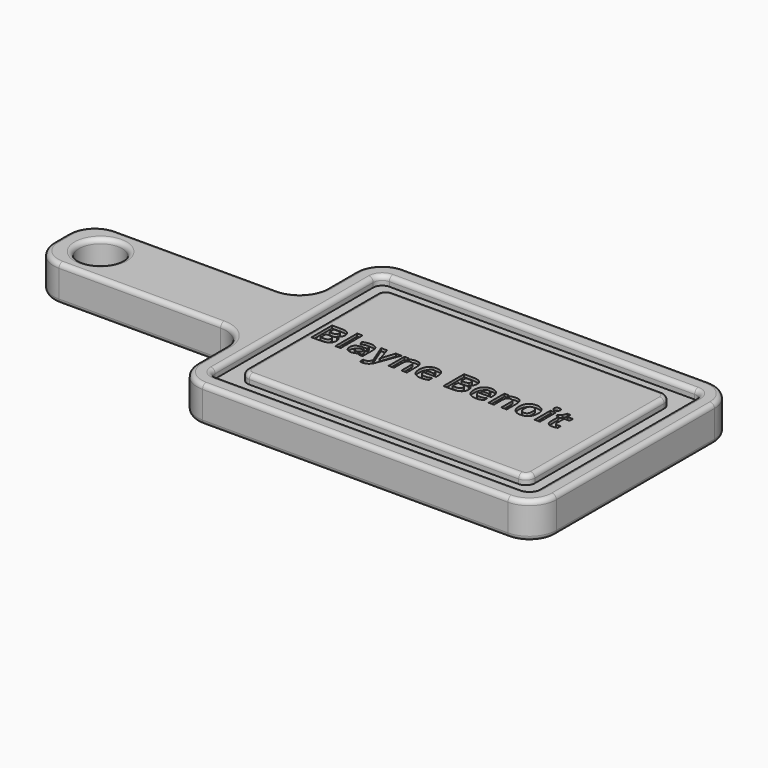
from build123d import *

# Parameters (mm, degrees)
F0_W         = 152.4
F0_H         = 50.8
F1_DEPTH     = 25.4
F2_R         = 15.24
F3_DEPTH     = 25.4
F5_DEPTH     = 6.35
F6_R         = 6.35
F7_R         = 19.05
F8_R         = 3.175
F9_TEXT_SIZE = 25.5139013453
F10_DEPTH    = 1.905


# Not quite as in the source:
# - Text() gives the source's letters only with a copy of the font that has no kerning and outlines rounded to 1/6400 em; it was checked with that copy


with BuildPart() as f1:
    # F0 (on Top) → F1 (new body)
    with BuildSketch(Plane.XY):
        Polygon((0, 63.5), (0, 0), (254, 0), (254, 177.8), (0, 177.8), (0, 114.3), align=None)
        with Locations((-76.2, 88.9)):
            Rectangle(F0_W, F0_H)
    extrude(amount=F1_DEPTH)

    # F2 (on face) → F3 (cut)
    with BuildSketch(Plane.XY.offset(25.4)):
        with Locations((-124.2342218757, 88.9)):
            Circle(F2_R)
    extrude(amount=-F3_DEPTH, mode=Mode.SUBTRACT)

    # F4 (on face) → F5 (cut)
    with BuildSketch(Plane.XY.offset(25.4)):
        Polygon((12.7, 38.1), (12.7, 12.7), (241.3, 12.7), (241.3, 165.1), (12.7, 165.1), (12.7, 88.9), align=None)
        Polygon((25.4, 38.1), (25.4, 88.9), (25.4, 152.4), (228.6, 152.4), (228.6, 25.4), (25.4, 25.4), align=None, mode=Mode.SUBTRACT)
    extrude(amount=-F5_DEPTH, mode=Mode.SUBTRACT)

    # F6
    f6_edges = [f1.edges().sort_by_distance(p)[0] for p in [
        (12.7, 165.1, 22.225),
        (241.3, 165.1, 22.225),
        (241.3, 12.7, 22.225),
        (12.7, 12.7, 22.225),
        (228.6, 152.4, 22.225),
        (228.6, 25.4, 22.225),
        (25.4, 152.4, 22.225),
        (25.4, 25.4, 22.225),
    ]]
    fillet(f6_edges, radius=F6_R)

    # F7
    f7_edges = [f1.edges().sort_by_distance(p)[0] for p in [
        (254, 0, 12.7),
        (-152.4, 63.5, 12.7),
        (0, 0, 12.7),
        (254, 177.8, 12.7),
        (0, 177.8, 12.7),
        (-152.4, 114.3, 12.7),
        (0, 114.3, 12.7),
        (0, 63.5, 12.7),
    ]]
    fillet(f7_edges, radius=F7_R)

    # F8
    f8_edges = [f1.edges().sort_by_distance(p)[0] for p in [
        (127, 152.4, 25.4),
        (27.259872, 150.540128, 25.4),
        (226.740128, 150.540128, 25.4),
        (25.4, 88.9, 25.4),
        (228.6, 88.9, 25.4),
        (27.259872, 27.259872, 25.4),
        (226.740128, 27.259872, 25.4),
        (127, 25.4, 25.4),
        (0, 31.75, 25.4),
        (-5.579616, 57.920384, 25.4),
        (5.579616, 5.579616, 25.4),
        (-76.2, 63.5, 25.4),
        (127, 0, 25.4),
        (-146.820384, 69.079616, 25.4),
        (248.420384, 5.579616, 25.4),
        (-152.4, 88.9, 25.4),
        (254, 88.9, 25.4),
        (-146.820384, 108.720384, 25.4),
        (248.420384, 172.220384, 25.4),
        (-76.2, 114.3, 25.4),
        (127, 177.8, 25.4),
        (-5.579616, 119.879616, 25.4),
        (5.579616, 172.220384, 25.4),
        (0, 146.05, 25.4),
        (127, 12.7, 25.4),
        (14.559872, 14.559872, 25.4),
        (239.440128, 14.559872, 25.4),
        (12.7, 88.9, 25.4),
        (241.3, 88.9, 25.4),
        (14.559872, 163.240128, 25.4),
        (239.440128, 163.240128, 25.4),
        (127, 165.1, 25.4),
        (-139.474222, 88.9, 25.4),
        (0, 31.75, 0),
        (-5.579616, 57.920384, 0),
        (5.579616, 5.579616, 0),
        (-76.2, 63.5, 0),
        (127, 0, 0),
        (-146.820384, 69.079616, 0),
        (248.420384, 5.579616, 0),
        (-152.4, 88.9, 0),
        (254, 88.9, 0),
        (-146.820384, 108.720384, 0),
        (248.420384, 172.220384, 0),
        (-76.2, 114.3, 0),
        (127, 177.8, 0),
        (-5.579616, 119.879616, 0),
        (5.579616, 172.220384, 0),
        (0, 146.05, 0),
        (-139.474222, 88.9, 0),
    ]]
    fillet(f8_edges, radius=F8_R)

    # F9 (on face) → F10 (cut)
    with BuildSketch(Plane.XY.offset(25.4)):
        with Locations((28.575, 81.4646694779)):
            Text('Blayne Benoit', F9_TEXT_SIZE, font='Open Sans', font_style=FontStyle.BOLD, text_align=(TextAlign.LEFT, TextAlign.BOTTOM))
    extrude(amount=-F10_DEPTH, mode=Mode.SUBTRACT)


solid = f1.part
